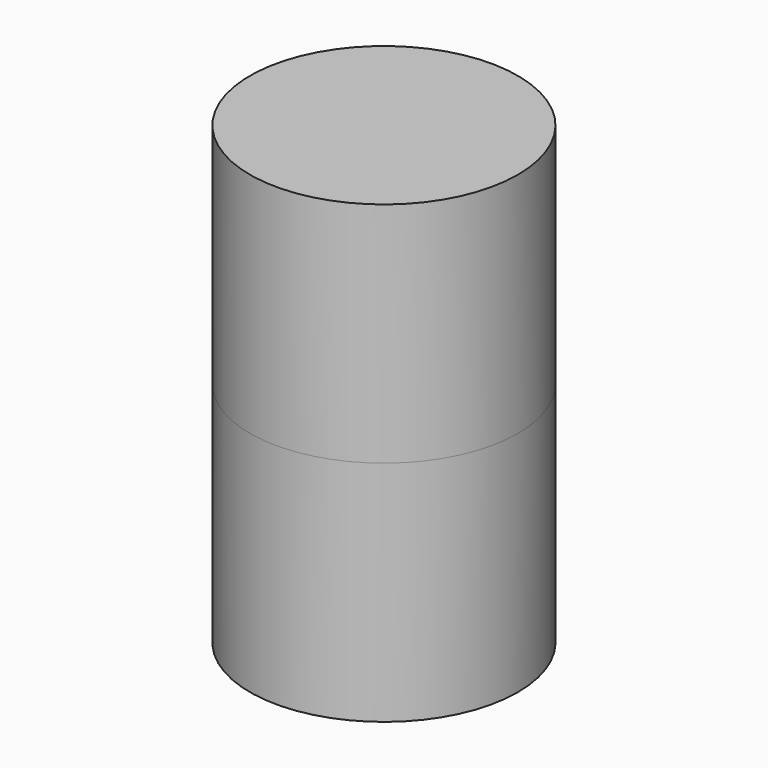
from build123d import *

# Parameters (mm, degrees)
F0_R     = 20
F1_DEPTH = 34
F2_DEPTH = 34


# Not quite as in the source:
# - a feature of the source that left no trace in its solid (it failed there, or was rolled back) is left out


with BuildPart() as f1:
    # F0 (on Top) → F1 (new body)
    with BuildSketch(Plane.XY):
        Circle(F0_R)
    extrude(amount=-F1_DEPTH)


with BuildPart() as f2:
    # F2 (new): a face of the model
    f2_faces = [f1.part.faces().sort_by_distance(p)[0] for p in [
        (0, 0, 0),
    ]]
    extrude(f2_faces, amount=F2_DEPTH)


solid = Compound([f1.part, f2.part])
